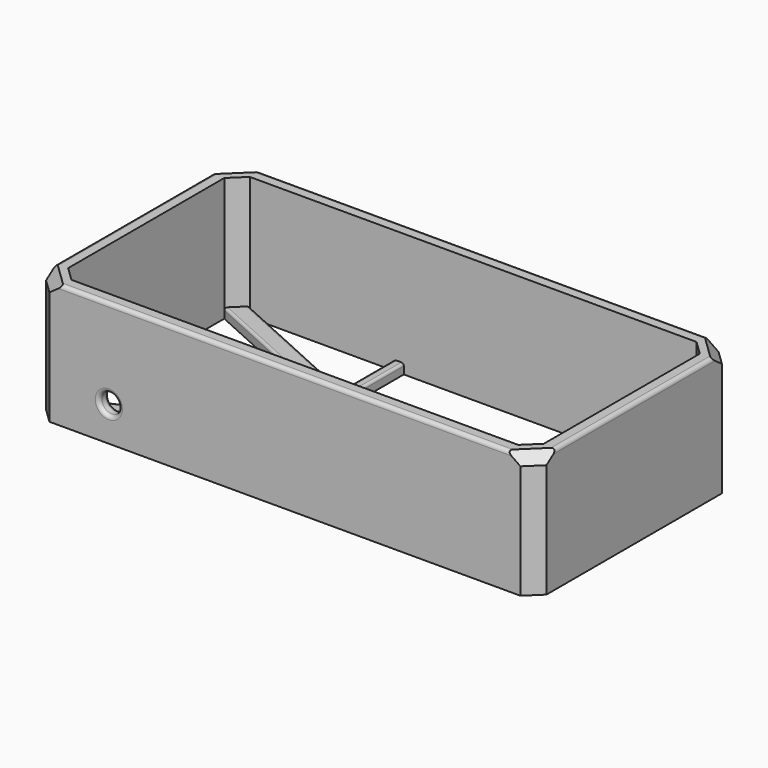
from build123d import *

# Parameters (mm, degrees)
F1_DEPTH = 25
F2_R     = 2
F3_DEPTH = 25
F4_SIZE  = 2
F5_DEPTH = 2
F6_R     = 0.5
F7_R     = 0.75


with BuildPart() as f1:
    # F0 (on Top) → F1 (new body)
    with BuildSketch(Plane.XY):
        Polygon((47.5420507878, 25), (-47.5420507878, 25), (-50.5, 22.1415455767), (-50.5, -22.1415455767), (-47.5420507878, -25), (47.5420507878, -25), (50.5, -22.1415455767), (50.5, 22.1415455767), align=None)
        Polygon((-48, 19.6920558339), (-45.092561045, 22.5), (-16, 22.5), (-14, 22.5), (45.092561045, 22.5), (48, 19.6920558339), (48, -19.6920558339), (45.092561045, -22.5), (-45.092561045, -22.5), (-48, -19.6920558339), (-48, 1.5), (-48, 3.5), align=None, mode=Mode.SUBTRACT)
    extrude(amount=F1_DEPTH)

    # F2 (on face) → F3 (cut)
    with BuildSketch(Plane.XZ.offset(25)):
        with Locations((-35.5420507878, 7)):
            Circle(F2_R)
    extrude(amount=-F3_DEPTH, mode=Mode.SUBTRACT)

    # F4
    f4_edges = [f1.edges().sort_by_distance(p)[0] for p in [
        (-49.021025, -23.570773, 25),
        (49.021025, -23.570773, 25),
        (49.021025, 23.570773, 25),
        (-49.021025, 23.570773, 25),
    ]]
    chamfer(f4_edges, length=F4_SIZE)

    # F7
    f7_edges = [f1.edges().sort_by_distance(p)[0] for p in [
        (0, -25, 25),
        (-50.5, 0, 25),
        (0, 25, 25),
        (50.5, 0, 25),
        (-37.542051, -25, 7),
        (-33.542051, -23.75, 7),
        (-37.542051, -22.5, 7),
    ]]
    fillet(f7_edges, radius=F7_R)


with BuildPart() as f5:
    # F0 (on Top) → F5 (new body)
    with BuildSketch(Plane.XY):
        Polygon((-16, 9.3144678137), (-45.092561045, 22.5), (-48, 19.6920558339), (-16, 5.1887940101), align=None)
        Polygon((-14, 22.5), (-16, 22.5), (-16, 9.3144678137), (-16, 5.1887940101), (-16, 3.5), (-48, 3.5), (-48, 1.5), (-14, 1.5), (-14, 4.2823401461), (-14, 8.4080139497), align=None)
        Polygon((48, 19.6920558339), (45.092561045, 22.5), (0, 2.0628369018), (-14, 8.4080139497), (-14, 4.2823401461), (-4.5514437827, 0), (-48, -19.6920558339), (-45.092561045, -22.5), (0, -2.0628369018), (45.092561045, -22.5), (48, -19.6920558339), (4.5514437827, 0), align=None)
    extrude(amount=F5_DEPTH)

    # F6
    f6_edges = [f5.edges().sort_by_distance(p)[0] for p in [
        (-30.546281, 15.907234, 2),
        (-32, 12.440425, 2),
        (-32, 3.5, 2),
        (-31, 1.5, 2),
        (-14, 2.89117, 2),
        (-9.275722, 2.14117, 2),
        (22.546281, 12.281418, 2),
        (26.275722, 9.846028, 2),
        (22.546281, -12.281418, 2),
        (26.275722, -9.846028, 2),
        (-22.546281, -12.281418, 2),
        (-26.275722, -9.846028, 2),
        (-14, 15.454007, 2),
        (-16, 15.907234, 2),
        (-7, 5.235425, 2),
    ]]
    fillet(f6_edges, radius=F6_R)


solid = Compound([f1.part, f5.part])
